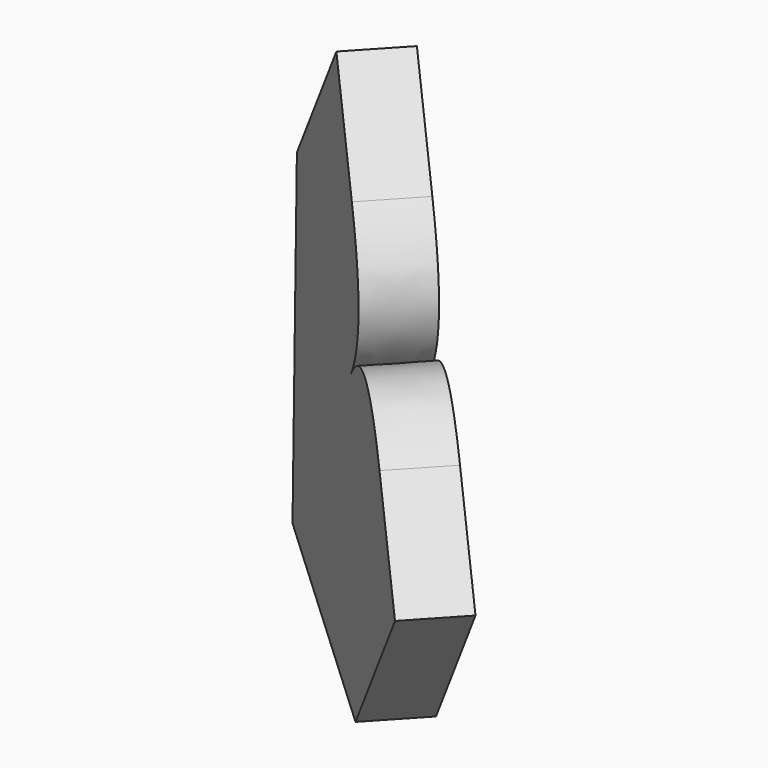
from build123d import *

# Parameters (mm, degrees)
F1_DEPTH    = 11.62886
F2_T1_DEPTH = 111.62886
F4_ANGLE    = -90


# Not quite as in the source:
# - a fillet or chamfer that OpenCascade refuses, or shapes differently, is made with other operations: its cross-section is extruded or revolved along the edge and cut away or added


with BuildPart() as f1:
    # F0 (on Top) → F1 (new body)
    with BuildSketch(Plane.XY):
        Polygon((45.4364679754, 42.3810482025), (0, 0), (98.7063497305, 0), (98.7063497305, 42.3810482025), align=None)
    extrude(amount=F1_DEPTH)

    # F2: fillet of radius 20 on 1 edges, made by hand

    # F2_s2 → F2_t1 (cut)
    with BuildSketch(Plane.XY.offset(-50)):
        with BuildLine():
            add(Edge.make_bspline(
                [(78.7063497305, 0), (98.7063497305, 0), (98.7063497305, 20)],
                knots=[0, 0, 0, 1, 1, 1], degree=2, weights=[1, 1, 1]))
            Line((98.7063497305, 20), (98.7063497305, 0))
            Line((98.7063497305, 0), (78.7063497305, 0))
        make_face()
    extrude(amount=F2_T1_DEPTH, mode=Mode.SUBTRACT)

    # F3: F1 across plane


with BuildPart() as f1_1:
    add(f1.part)
    add(f1.part.mirror(Plane.XZ))


with BuildPart() as f1_2:
    # F4: moved
    add(f1_1.part.rotate(Axis((22.7182339877, -21.1905241013, 11.62886), (-0.7312665459, 0.6820918111, 0)), F4_ANGLE))


solid = f1_2.part
